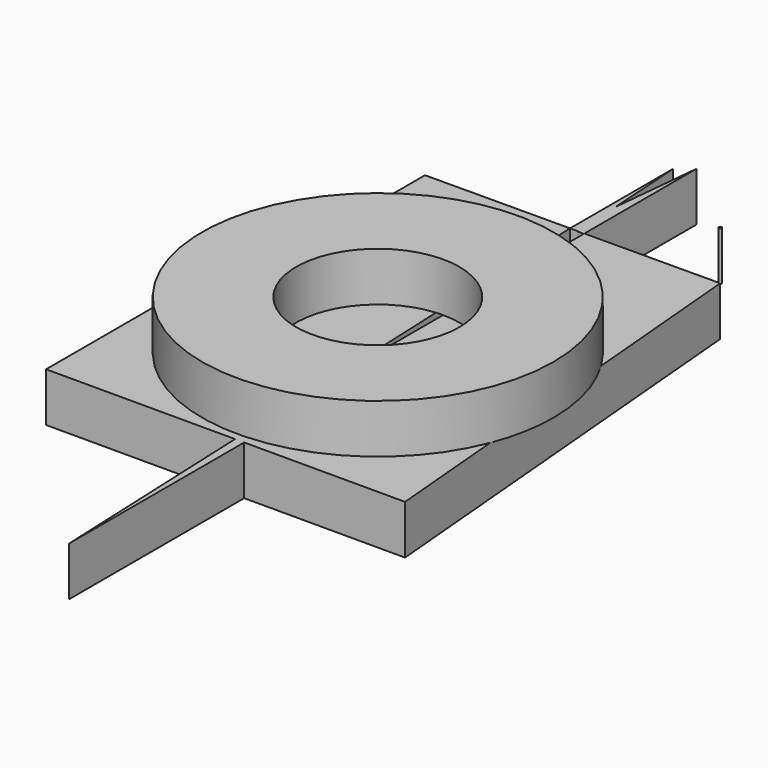
from build123d import *

# Parameters (mm, degrees)
F1_DEPTH = 25.4
F2_R     = 0.6873607635
F2_R_2   = 90.9704794281
F2_R_3   = 42.2453138018
F3_DEPTH = 25.4


with BuildPart() as f1:
    # F0 (on Top) → F1 (new body)
    with BuildSketch(Plane.XY):
        Polygon((0, 89.7069421623), (0, 0), (-1.810804775, 0), (2.1516823224, -95.0307697058), (6.8773888052, -95.0307697058), (6.8773888052, -13.3527815342), align=None)
        Polygon((2.1516823224, -95.0307697058), (-1.810804775, 0), (-95.6487208605, 0), (-95.6487208605, -95.0307697058), align=None)
        Polygon((-95.6487208605, 0), (-1.810804775, 0), (-5.859600791, 97.1006825566), (-82.1735113859, 97.1006825566), (-95.6487208605, 97.1006825566), align=None)
        Polygon((0, 97.1006825566), (0, 89.7069421623), (6.8773888052, -13.3527815342), (6.8773888052, -95.0307697058), (90.1318565011, -95.0307697058), (70.0762048364, 133.9463293552), (0, 133.6299567875), (0, 133.2589685917), align=None)
        Polygon((-82.1735113859, 97.1006825566), (-5.859600791, 97.1006825566), (-7.3672886938, 133.2589685917), (-82.1735113859, 133.2589685917), align=None)
        Polygon((6.8773888052, -95.0307697058), (2.1516823224, -95.0307697058), (6.8773888052, -208.3655297756), align=None)
        Polygon((-7.3672886938, 133.5966957391), (-7.3672886938, 133.2589685917), (-7.3332104262, 133.596849592), align=None)
        Polygon((-82.1735113859, 133.2589685917), (-7.3672886938, 133.2589685917), (-7.3672886938, 133.5966957391), align=None)
        Polygon((-2.9063169225, 133.2589685917), (0, 133.2589685917), (0, 133.6299567875), (-2.9301909404, 133.6167278743), align=None)
        Polygon((-7.3672886938, 133.5966957391), (-7.3332104262, 133.596849592), (-4.6826064537, 159.8771973232), (-7.3672886938, 200.1079618931), align=None)
        Polygon((-4.6826064537, 159.8771973232), (-7.3332104262, 133.596849592), (-2.9301909404, 133.6167278743), align=None)
        Polygon((-2.9301909404, 133.6167278743), (0, 133.6299567875), (0, 206.3045501709), (-4.6826064537, 159.8771973232), align=None)
    extrude(amount=F1_DEPTH)

    # F2 (on face) → F3 (join)
    with BuildSketch(Plane.XY.offset(25.4)):
        with Locations((70.0762048364, 133.9463293552)):
            Circle(F2_R)
        Circle(F2_R_2)
        Circle(F2_R_3, mode=Mode.SUBTRACT)
    extrude(amount=F3_DEPTH)


solid = f1.part
